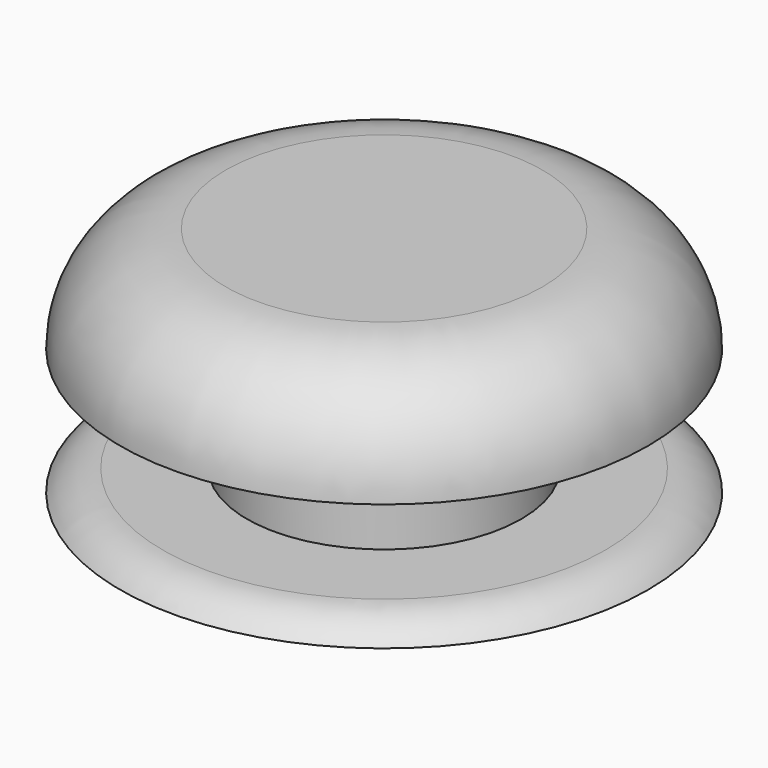
from build123d import *

# Parameters (mm, degrees)
F0_R     = 25
F0_R_2   = 13
F0_R_3   = 11
F0_R_4   = 8
F0_R_5   = 5
F0_R_6   = 3
F1_DEPTH = 2
F2_DEPTH = 10
F3_DEPTH = 4
F5_DEPTH = 20
F6_DEPTH = 20
F7_DEPTH = 10
F8_R     = 9.99999
F9_START = 15
F9_DEPTH = 5


# Not quite as in the source:
# - a fillet or chamfer that OpenCascade refuses, or shapes differently, is made with other operations: its cross-section is extruded or revolved along the edge and cut away or added
# - a fillet or chamfer is up to 0.001 mm smaller than in the source, because OpenCascade refuses the exact size


with BuildPart() as f1:
    # F0 (on Top) → F1 (new body)
    with BuildSketch(Plane.XY):
        Circle(F0_R)
        Circle(F0_R_2, mode=Mode.SUBTRACT)
        Circle(F0_R_2)
        Circle(F0_R_3, mode=Mode.SUBTRACT)
        Circle(F0_R_3)
        Circle(F0_R_4, mode=Mode.SUBTRACT)
        Circle(F0_R_4)
        Circle(F0_R_5, mode=Mode.SUBTRACT)
        Circle(F0_R_5)
        Circle(F0_R_6, mode=Mode.SUBTRACT)
    extrude(amount=-F1_DEPTH)

    # F0 (on Top) → F2 (join)
    with BuildSketch(Plane.XY):
        Circle(F0_R_2)
        Circle(F0_R_3, mode=Mode.SUBTRACT)
    extrude(amount=F2_DEPTH)

    # F0 (on Top) → F3 (join)
    with BuildSketch(Plane.XY):
        Circle(F0_R_4)
        Circle(F0_R_5, mode=Mode.SUBTRACT)
    extrude(amount=F3_DEPTH)

    # F4: fillet of radius 5.08 on 1 edges, made by hand

    # F4_s1 → F4_t2 (revolve, cut)
    with BuildSketch(Plane.XZ):
        with BuildLine():
            ThreePointArc((25, -2), (23.2140835586, -0.5273743839), (20.9601980247, 0))
            Line((20.9601980247, 0), (25, 0))
            Line((25, 0), (25, -2))
        make_face()
    revolve(axis=Axis((0, 0, 0), (0, 0, 1)), mode=Mode.SUBTRACT)


with BuildPart() as f5:
    # F0 (on Top) → F5 (new body)
    with BuildSketch(Plane.XY):
        Circle(F0_R_5)
        Circle(F0_R_6, mode=Mode.SUBTRACT)
    extrude(amount=F5_DEPTH)

    # F0 (on Top) → F6 (join)
    with BuildSketch(Plane.XY):
        Circle(F0_R)
        Circle(F0_R_2, mode=Mode.SUBTRACT)
        Circle(F0_R_2)
        Circle(F0_R_3, mode=Mode.SUBTRACT)
        Circle(F0_R_3)
        Circle(F0_R_4, mode=Mode.SUBTRACT)
        Circle(F0_R_4)
        Circle(F0_R_5, mode=Mode.SUBTRACT)
    extrude(amount=F6_DEPTH)

    # F0 (on Top) → F7 (cut)
    with BuildSketch(Plane.XY):
        Circle(F0_R)
        Circle(F0_R_2, mode=Mode.SUBTRACT)
        Circle(F0_R_2)
        Circle(F0_R_3, mode=Mode.SUBTRACT)
        Circle(F0_R_3)
        Circle(F0_R_4, mode=Mode.SUBTRACT)
        Circle(F0_R_4)
        Circle(F0_R_5, mode=Mode.SUBTRACT)
    extrude(amount=F7_DEPTH, mode=Mode.SUBTRACT)

    # F8 (radius 10 in the source; OpenCascade refuses exactly that, so slightly less here)
    f8_edges = [f5.edges().sort_by_distance(p)[0] for p in [
        (-25, 0, 20),
    ]]
    fillet(f8_edges, radius=F8_R)

    # F0 (on Top) → F9 (join)
    with BuildSketch(Plane.XY.offset(F9_START)):
        Circle(F0_R_6)
    extrude(amount=F9_DEPTH)


solid = Compound([f1.part, f5.part])
